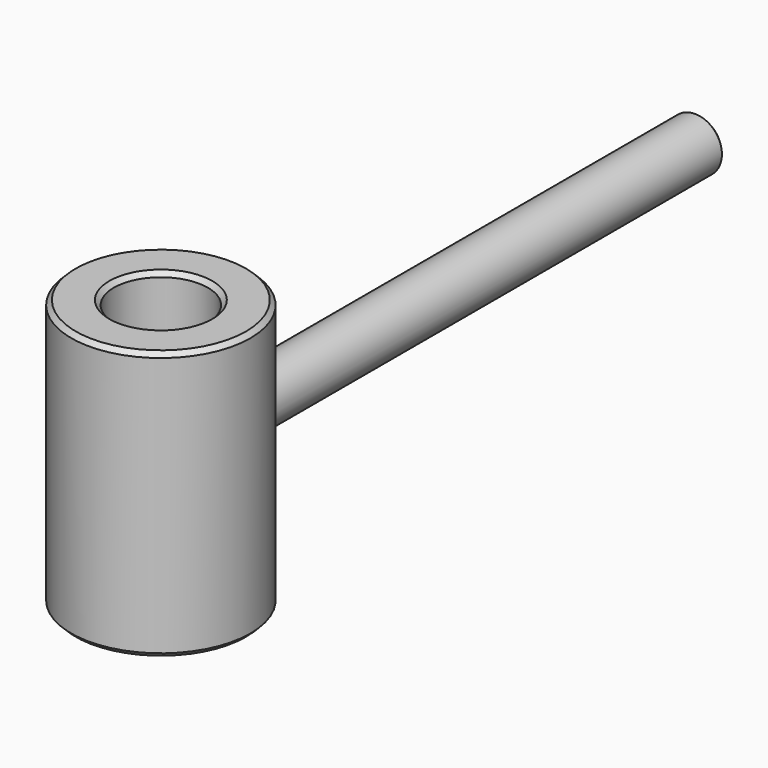
from build123d import *

# Parameters (mm, degrees)
F0_R     = 20
F1_DEPTH = 30
F3_D     = 21
F5_R     = 6
F7_SIZE  = 1


with BuildPart() as f1:
    # F0 (on Top) → F1 (new body, symmetric)
    with BuildSketch(Plane.XY):
        Circle(F0_R)
    extrude(amount=F1_DEPTH, both=True)

    # F3 (through all)
    with Locations(Plane.XY.offset(30)):
        with Locations((0, 0)):
            Hole(F3_D / 2)

    # F5 (on offset) → F6 (join, up to the next surface of F1)
    with BuildSketch(Plane.XZ.offset(-150)):
        Circle(F5_R)
    extrude(until=Until.NEXT)

    # F7
    f7_edges = [f1.edges().sort_by_distance(p)[0] for p in [
        (-6, 150, 0),
        (-20, 0, 30),
        (-20, 0, -30),
        (-10.5, 0, 30),
        (-10.5, 0, -30),
    ]]
    chamfer(f7_edges, length=F7_SIZE)


solid = f1.part
